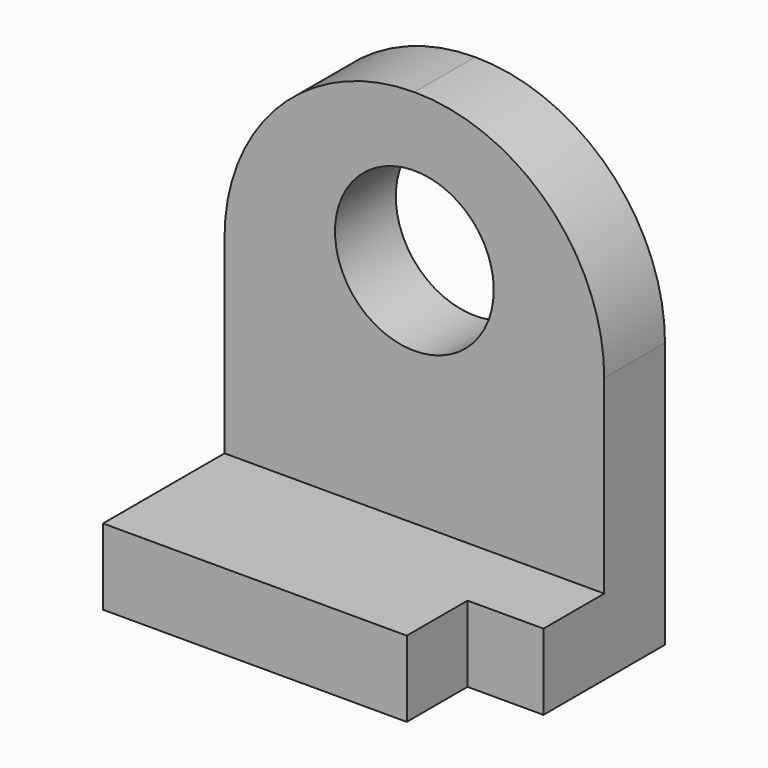
from build123d import *

# Parameters (mm, degrees)
F1_DEPTH = 25.4
F2_W     = 127
F2_H     = 25.4
F3_DEPTH = 127
F4_R     = 63.5
F5_R     = 63.49999
F6_R     = 26.5461499869
F7_DEPTH = 25.401


# Not quite as in the source:
# - a fillet or chamfer is up to 0.001 mm smaller than in the source, because OpenCascade refuses the exact size


with BuildPart() as f1:
    # F0 (on Top) → F1 (new body)
    with BuildSketch(Plane.XY):
        Polygon((63.5, -12.7), (63.5, 38.1), (-63.5, 38.1), (-63.5, -38.1), (38.1, -38.1), (38.1, -12.7), align=None)
    extrude(amount=F1_DEPTH)

    # F2 (on face) → F3 (join)
    with BuildSketch(Plane.XY.offset(25.4)):
        with Locations((0, 25.4)):
            Rectangle(F2_W, F2_H)
    extrude(amount=F3_DEPTH)

    # F4
    f4_edges = [f1.edges().sort_by_distance(p)[0] for p in [
        (63.5, 25.4, 152.4),
    ]]
    fillet(f4_edges, radius=F4_R)

    # F5 (radius 63.5 in the source; OpenCascade refuses exactly that, so slightly less here)
    f5_edges = [f1.edges().sort_by_distance(p)[0] for p in [
        (-63.5, 25.4, 152.4),
    ]]
    fillet(f5_edges, radius=F5_R)

    # F6 (on face) → F7 (cut, through all)
    with BuildSketch(Plane.XZ.offset(-12.7)):
        with Locations((0, 102.7461499869)):
            Circle(F6_R)
    extrude(amount=-F7_DEPTH, mode=Mode.SUBTRACT)


solid = f1.part
